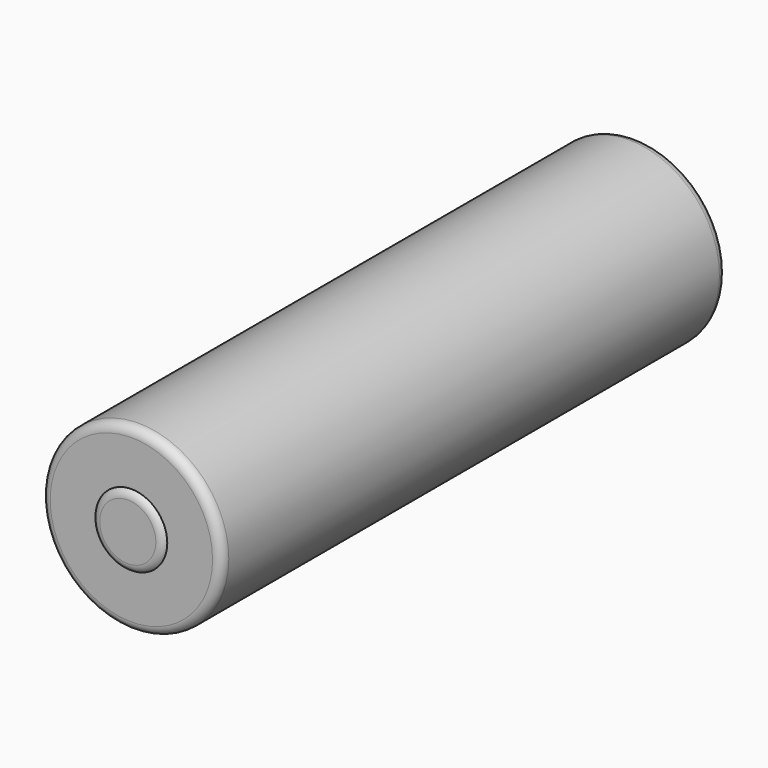
from build123d import *

# Parameters (mm, degrees)
F0_R     = 10
F1_DEPTH = 70
F2_R     = 1
F3_R     = 3.9775912989
F4_DEPTH = 0.5


# Not quite as in the source:
# - a fillet or chamfer that OpenCascade refuses, or shapes differently, is made with other operations: its cross-section is extruded or revolved along the edge and cut away or added


with BuildPart() as f1:
    # F0 (on Front) → F1 (new body)
    with BuildSketch(Plane.XZ):
        Circle(F0_R)
    extrude(amount=F1_DEPTH)

    # F2
    f2_edges = [f1.edges().sort_by_distance(p)[0] for p in [
        (-10, -70, 0),
        (-10, 0, 0),
    ]]
    fillet(f2_edges, radius=F2_R)

    # F3 (on face) → F4 (join)
    with BuildSketch(Plane.XZ.offset(70)):
        Circle(F3_R)
    extrude(amount=F4_DEPTH)

    # F5: fillet of radius 1 on 1 edges, made by hand

    # F5_s1 → F5_t2 (revolve, cut)
    with BuildSketch(Plane.XY):
        with BuildLine():
            ThreePointArc((3.9775912989, -70), (3.6115658951, -70.3660254038), (3.1115658951, -70.5))
            Line((3.1115658951, -70.5), (3.9775912989, -70.5))
            Line((3.9775912989, -70.5), (3.9775912989, -70))
        make_face()
    revolve(axis=Axis((0, -70.5, 0), (0, -1, 0)), mode=Mode.SUBTRACT)


solid = f1.part
